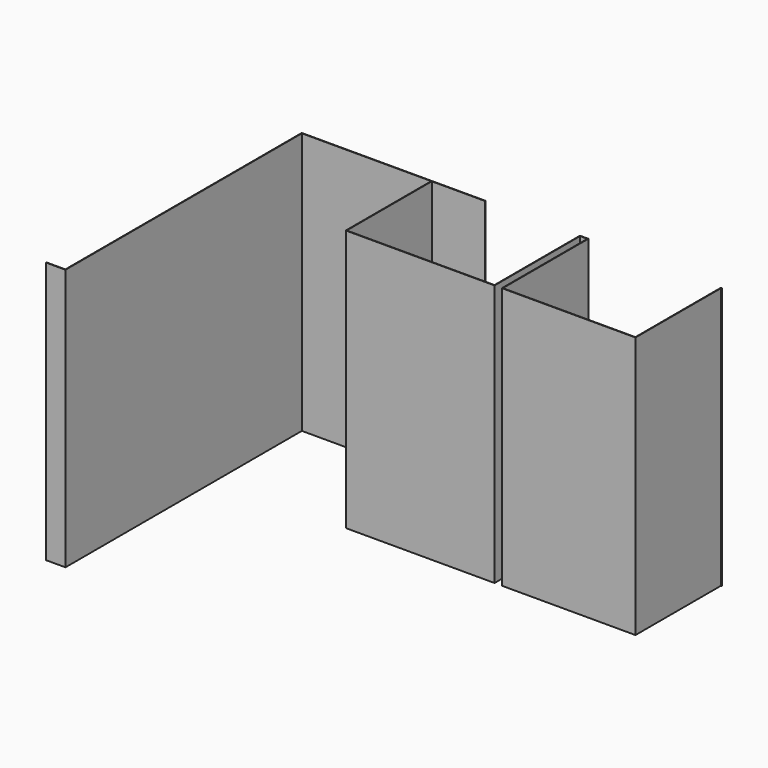
from build123d import *

# Parameters (mm, degrees)
F0_W     = 510
F0_H     = 5
F1_DEPTH = 2500


# Not quite as in the source:
# - a feature names something its author has since deleted; it is built from what else it names


with BuildPart() as f1:
    # F0 (on Top) → F1 (new body)
    with BuildSketch(Plane.XY):
        Polygon((867.7531446819, 942.2693800055), (-542.2468553181, 942.2693800055), (-542.2468553181, 1957.2693800055), (-542.2468553181, 1962.2693800055), (-1787.2468553181, 1962.2693800055), (-1787.2468553181, -857.7306199945), (-1967.2468553181, -857.7306199945), (-1967.2468553181, -862.7306199945), (-1782.2468553181, -862.7306199945), (-1782.2468553181, 1957.2693800055), (-547.2468553181, 1957.2693800055), (-547.2468553181, 937.2693800055), (872.7531446819, 937.2693800055), (872.7531446819, 1957.2693800055), (942.7531446819, 1957.2693800055), (942.7531446819, 937.2693800055), (2217.7531446819, 937.2693800055), (2217.7531446819, 1957.2693800055), (2222.7531446819, 1957.2693800055), (2222.7531446819, 1962.2693800055), (2212.7531446819, 1962.2693800055), (2212.7531446819, 942.2693800055), (947.7531446819, 942.2693800055), (947.7531446819, 1962.2693800055), (867.7531446819, 1962.2693800055), align=None)
        with Locations((-287.2468553181, 1959.7693800055)):
            Rectangle(F0_W, F0_H)
    extrude(amount=F1_DEPTH)


solid = f1.part
